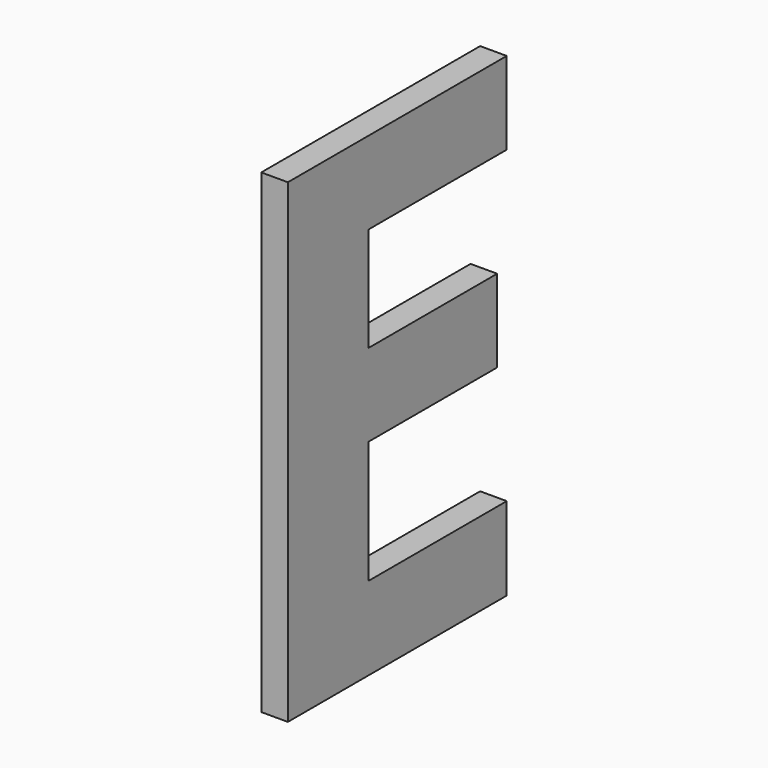
from build123d import *

# Parameters (mm, degrees)
F0_TEXT_SIZE = 635
F1_DEPTH     = 12.7


# Not quite as in the source:
# - Text() gives the source's letters only with a copy of the font that has no kerning and outlines rounded to 1/6400 em; it was checked with that copy


with BuildPart() as f1:
    # F0 (on Right) → F1 (new body, symmetric)
    with BuildSketch(Plane.YZ):
        with Locations((-318.0953125, 0)):
            Text('E', F0_TEXT_SIZE, font='Open Sans', font_style=FontStyle.BOLD, text_align=(TextAlign.LEFT, TextAlign.BOTTOM))
    extrude(amount=F1_DEPTH, both=True)


solid = f1.part
